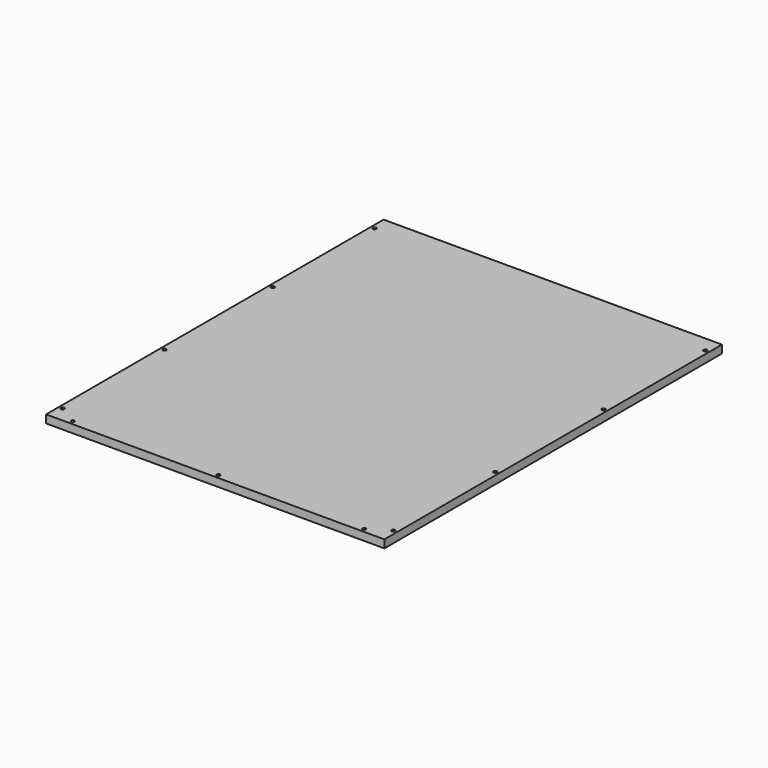
from build123d import *

# Parameters (mm, degrees)
F0_W           = 425
F0_H           = 530
F1_DEPTH       = 5
F3_D           = 4.4
F3_CBORE_D     = 8.25
F3_CBORE_DEPTH = 4


# Not quite as in the source:
# - a feature names something its author has since deleted; it is built from what else it names


with BuildPart() as f1:
    # F0 (on Top) → F1 (new body, symmetric)
    with BuildSketch(Plane.XY):
        Rectangle(F0_W, F0_H)
    extrude(amount=F1_DEPTH, both=True)

    # F3 (through all)
    with Locations(Plane(origin=(0, 0, -5), x_dir=(1, 0, 0), z_dir=(0, 0, -1))):
        with Locations((-207.75, 245), (-207.75, 85), (-207.75, -85), (-207.75, -245), (207.75, -245), (207.75, -85), (207.75, 85), (207.75, 245), (-183, 260), (0, 260), (183, 260)):
            CounterBoreHole(F3_D / 2, F3_CBORE_D / 2, F3_CBORE_DEPTH)


solid = f1.part
